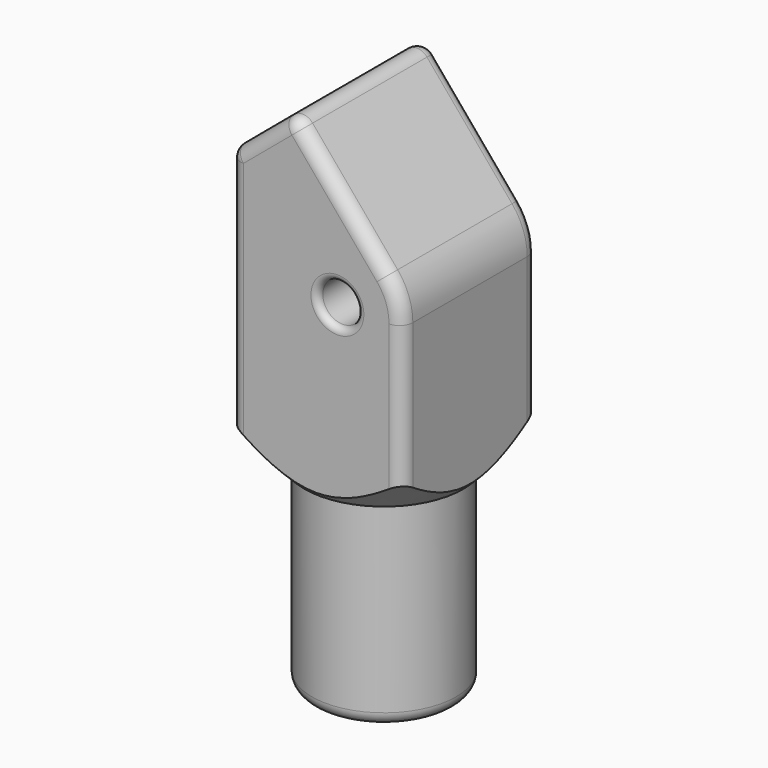
from build123d import *

# Parameters (mm, degrees)
F0_R      = 1.5
F1_DEPTH  = 12.8
F2_R      = 4.9
F3_R      = 1
F4_R      = 5.45
F5_DEPTH  = 15
F9_R      = 3.45
F10_DEPTH = 25
F11_R     = 0.99999
F12_R     = 0.5


# Not quite as in the source:
# - a fillet or chamfer is up to 0.001 mm smaller than in the source, because OpenCascade refuses the exact size


with BuildPart() as f1:
    # F0 (on Front) → F1 (new body)
    with BuildSketch(Plane.XZ):
        Polygon((-13, 0), (0, 0), (0, 15.2073059861), (-8.2170459353, 25), (-13, 20.9866250083), align=None)
        with Locations((-4.9, 13.4238518382)):
            Circle(F0_R, mode=Mode.SUBTRACT)
    extrude(amount=F1_DEPTH)

    # F2
    f2_edges = [f1.edges().sort_by_distance(p)[0] for p in [
        (0, -6.4, 15.207306),
    ]]
    fillet(f2_edges, radius=F2_R)

    # F3
    f3_edges = [f1.edges().sort_by_distance(p)[0] for p in [
        (-8.217046, -6.4, 25),
        (-13, -6.4, 20.986625),
    ]]
    fillet(f3_edges, radius=F3_R)

    # F4 (on face) → F5 (join)
    with BuildSketch(Plane(origin=(0, 0, 0), x_dir=(1, 0, 0), z_dir=(0, 0, -1))):
        with Locations((-6.5, 6.4)):
            Circle(F4_R)
    extrude(amount=F5_DEPTH)

    # F7 (on offset) → F8 (revolve, cut)
    with BuildSketch(Plane.YZ.offset(-6.5)):
        Polygon((-17.4, 0), (-12.4, 0), (-17.4, 5), align=None)
    revolve(axis=Axis((-6.5, -6.4, -7.3510144139), (0, 0, 1)), mode=Mode.SUBTRACT)

    # F9 (on face) → F10 (cut)
    with BuildSketch(Plane(origin=(0, 0, -15), x_dir=(1, 0, 0), z_dir=(0, 0, -1))):
        with Locations((-6.5, 6.4)):
            Circle(F9_R)
    extrude(amount=-F10_DEPTH, mode=Mode.SUBTRACT)

    # F11 (radius 1 in the source; OpenCascade refuses exactly that, so slightly less here)
    f11_edges = [f1.edges().sort_by_distance(p)[0] for p in [
        (-11.95, -6.4, -15),
        (-9.95, -6.4, -15),
        (-13, 0, 11.821134),
        (0, -12.8, 8.272902),
        (-9.95, -6.4, 10),
    ]]
    fillet(f11_edges, radius=F11_R)

    # F12
    f12_edges = [f1.edges().sort_by_distance(p)[0] for p in [
        (-6.4, -12.8, 13.423852),
        (-6.4, 0, 13.423852),
    ]]
    fillet(f12_edges, radius=F12_R)


solid = f1.part
